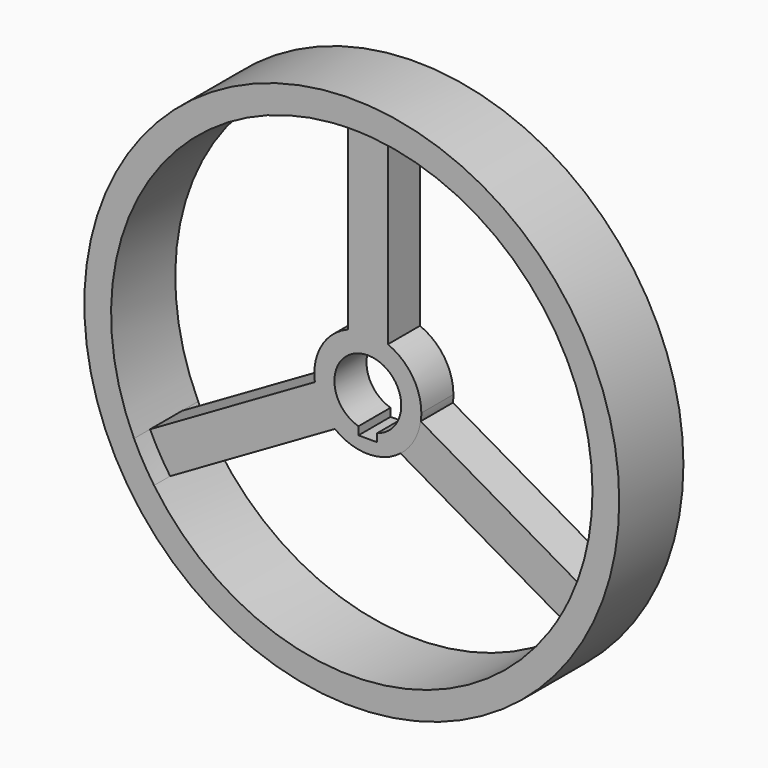
from build123d import *

# Parameters (mm, degrees)
F0_R     = 127
F1_DEPTH = 19.05
F2_DEPTH = 9.525
F3_DEPTH = 12.7
F4_DEPTH = 9.525
F5_DEPTH = 12.5848


with BuildPart() as f1:
    # F0 (on Front) → F1 (new body, symmetric)
    with BuildSketch(Plane.XZ):
        Circle(F0_R)
        with BuildLine():
            ThreePointArc((9.525, 113.902434), (84.122522, 77.381466), (114.3, 0))
            ThreePointArc((114.3, 0), (111.542974, -24.953054), (103.404901, -48.702325))
            ThreePointArc((103.404901, -48.702325), (98.986704, -57.15), (93.879901, -65.200109))
            ThreePointArc((93.879901, -65.200109), (0, -114.3), (-93.879901, -65.200109))
            ThreePointArc((-93.879901, -65.200109), (-98.986704, -57.15), (-103.404901, -48.702325))
            ThreePointArc((-103.404901, -48.702325), (-98.986704, 57.15), (-9.525, 113.902434))
            ThreePointArc((-9.525, 113.902434), (0, 114.3), (9.525, 113.902434))
        make_face(mode=Mode.SUBTRACT)
    extrude(amount=F1_DEPTH, both=True)

    # F0 (on Front) → F2 (join, symmetric)
    with BuildSketch(Plane.XZ):
        with BuildLine():
            Line((9.525, 23.54643), (9.525, 113.902434))
            ThreePointArc((9.525, 113.902434), (0, 114.3), (-9.525, 113.902434))
            Line((-9.525, 113.902434), (-9.525, 23.54643))
            ThreePointArc((-9.525, 23.54643), (0, 25.4), (9.525, 23.54643))
        make_face()
        with BuildLine():
            Line((-25.154307, -3.524323), (-103.404901, -48.702325))
            ThreePointArc((-103.404901, -48.702325), (-98.986704, -57.15), (-93.879901, -65.200109))
            Line((-93.879901, -65.200109), (-15.629307, -20.022107))
            ThreePointArc((-15.629307, -20.022107), (-21.997045, -12.7), (-25.154307, -3.524323))
        make_face()
        with BuildLine():
            ThreePointArc((93.879901, -65.200109), (98.986704, -57.15), (103.404901, -48.702325))
            Line((103.404901, -48.702325), (25.154307, -3.524323))
            ThreePointArc((25.154307, -3.524323), (21.997045, -12.7), (15.629307, -20.022107))
            Line((15.629307, -20.022107), (93.879901, -65.200109))
        make_face()
    extrude(amount=F2_DEPTH, both=True)

    # F0 (on Front) + F2_face (on face) → F3 (join, symmetric)
    with BuildSketch(Plane.XZ):
        Circle(F0_R)
        with BuildLine():
            ThreePointArc((9.525, 113.902434), (84.122522, 77.381466), (114.3, 0))
            ThreePointArc((114.3, 0), (111.542974, -24.953054), (103.404901, -48.702325))
            ThreePointArc((103.404901, -48.702325), (98.986704, -57.15), (93.879901, -65.200109))
            ThreePointArc((93.879901, -65.200109), (0, -114.3), (-93.879901, -65.200109))
            ThreePointArc((-93.879901, -65.200109), (-98.986704, -57.15), (-103.404901, -48.702325))
            ThreePointArc((-103.404901, -48.702325), (-98.986704, 57.15), (-9.525, 113.902434))
            ThreePointArc((-9.525, 113.902434), (0, 114.3), (9.525, 113.902434))
        make_face(mode=Mode.SUBTRACT)
    with BuildSketch(Plane(origin=(60.169627, -9.525, -34.73895), x_dir=(1, 0, 0), z_dir=(0, -1, 0))):
        with BuildLine():
            ThreePointArc((-35.01532, 31.214627), (-38.172581, 22.03895), (-44.54032, 14.716843))
            Line((-44.54032, 14.716843), (33.710274, -30.461159))
            ThreePointArc((33.710274, -30.461159), (38.817077, -22.41105), (43.235274, -13.963375))
            Line((43.235274, -13.963375), (-35.01532, 31.214627))
        make_face()
    extrude(amount=F3_DEPTH, both=True)

    # F0 (on Front) → F4 (join, symmetric)
    with BuildSketch(Plane.XZ):
        with BuildLine():
            ThreePointArc((25.4, 0), (21.060567, 14.199032), (9.525, 23.54643))
            ThreePointArc((9.525, 23.54643), (0, 25.4), (-9.525, 23.54643))
            ThreePointArc((-9.525, 23.54643), (-21.997045, 12.7), (-25.154307, -3.524323))
            ThreePointArc((-25.154307, -3.524323), (-21.997045, -12.7), (-15.629307, -20.022107))
            ThreePointArc((-15.629307, -20.022107), (0, -25.4), (15.629307, -20.022107))
            ThreePointArc((15.629307, -20.022107), (21.997045, -12.7), (25.154307, -3.524323))
            ThreePointArc((25.154307, -3.524323), (25.338502, -1.766438), (25.4, 0))
        make_face()
        with BuildLine():
            ThreePointArc((-4.445, -15.24), (0, 15.875), (4.445, -15.24))
            Line((4.445, -15.24), (4.445, -19.05))
            Line((4.445, -19.05), (-4.445, -19.05))
            Line((-4.445, -19.05), (-4.445, -15.24))
        make_face(mode=Mode.SUBTRACT)
    extrude(amount=F4_DEPTH, both=True)

    # F5 (cut): a face of the model
    f5_faces = [f1.faces().sort_by_distance(p)[0] for p in [
        (60.169627, -22.225, -34.73895),
    ]]
    extrude(f5_faces, amount=-F5_DEPTH, mode=Mode.SUBTRACT)


solid = f1.part
